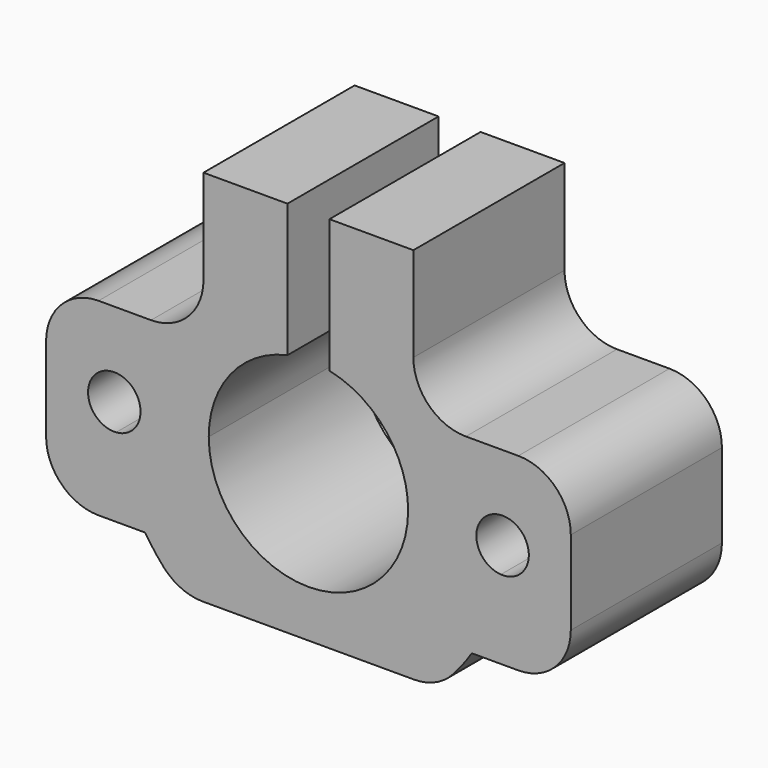
from build123d import *

# Parameters (mm, degrees)
F1_DEPTH = 18
F2_R     = 5


with BuildPart() as f1:
    # F0 (on Front) → F1 (new body)
    with BuildSketch(Plane.XZ):
        with BuildLine():
            ThreePointArc((12.0933866224, -14), (13.9727608958, -12.1248485743), (15.5643824163, -10))
            Line((15.5643824163, -10), (-15.5643824163, -10))
            ThreePointArc((-15.5643824163, -10), (-13.9727608958, -12.1248485743), (-12.0933866224, -14))
            Line((-12.0933866224, -14), (12.0933866224, -14))
        make_face()
        with BuildLine():
            Line((25, 8), (16.6808273176, 8))
            ThreePointArc((16.6808273176, 8), (17.7210793132, 5.311623855), (18.3310810811, 2.4942867515))
            ThreePointArc((18.3310810811, 2.4942867515), (20.2070006887, 1.8265127015), (21, 0))
            ThreePointArc((21, 0), (20.2070006887, -1.8265127015), (18.3310810811, -2.4942867515))
            ThreePointArc((18.3310810811, -2.4942867515), (17.358270198, -6.3984729219), (15.5643824163, -10))
            Line((15.5643824163, -10), (25, -10))
            Line((25, -10), (25, 8))
        make_face()
        with BuildLine():
            Line((2, 22), (2, 18.3915741577))
            ThreePointArc((2, 18.3915741577), (6.1642723241, 17.4428136123), (10, 15.5643824163))
            Line((10, 15.5643824163), (10, 22))
            Line((10, 22), (2, 22))
        make_face()
        with BuildLine():
            ThreePointArc((-10, 15.5643824163), (-6.1642723241, 17.4428136123), (-2, 18.3915741577))
            Line((-2, 18.3915741577), (-2, 22))
            Line((-2, 22), (-10, 22))
            Line((-10, 22), (-10, 15.5643824163))
        make_face()
        with BuildLine():
            ThreePointArc((-18.3310810811, 2.4942867515), (-17.7210793132, 5.311623855), (-16.6808273176, 8))
            Line((-16.6808273176, 8), (-25, 8))
            Line((-25, 8), (-25, -10))
            Line((-25, -10), (-15.5643824163, -10))
            ThreePointArc((-15.5643824163, -10), (-17.358270198, -6.3984729219), (-18.3310810811, -2.4942867515))
            ThreePointArc((-18.3310810811, -2.4942867515), (-21, 0), (-18.3310810811, 2.4942867515))
        make_face()
        with BuildLine():
            ThreePointArc((2, 9.2870878105), (3.6194093636, 8.7835002054), (5.123475383, 8))
            Line((5.123475383, 8), (10, 8))
            Line((10, 8), (10, 15.5643824163))
            ThreePointArc((10, 15.5643824163), (6.1642723241, 17.4428136123), (2, 18.3915741577))
            Line((2, 18.3915741577), (2, 9.2870878105))
        make_face()
        with BuildLine():
            Line((-10, 8), (-5.123475383, 8))
            ThreePointArc((-5.123475383, 8), (-3.6194093636, 8.7835002054), (-2, 9.2870878105))
            Line((-2, 9.2870878105), (-2, 18.3915741577))
            ThreePointArc((-2, 18.3915741577), (-6.1642723241, 17.4428136123), (-10, 15.5643824163))
            Line((-10, 15.5643824163), (-10, 8))
        make_face()
        with BuildLine():
            Line((10, 0), (9.5, 0))
            ThreePointArc((9.5, 0), (0, -9.5), (-9.5, 0))
            Line((-9.5, 0), (-10, 0))
            Line((-10, 0), (-10, 8))
            Line((-10, 8), (-16.6808273176, 8))
            ThreePointArc((-16.6808273176, 8), (-17.7210793132, 5.311623855), (-18.3310810811, 2.4942867515))
            ThreePointArc((-18.3310810811, 2.4942867515), (-16.6734872985, 1.7070006887), (-16, 0))
            ThreePointArc((-16, 0), (-16.6734872985, -1.7070006887), (-18.3310810811, -2.4942867515))
            ThreePointArc((-18.3310810811, -2.4942867515), (-17.358270198, -6.3984729219), (-15.5643824163, -10))
            Line((-15.5643824163, -10), (15.5643824163, -10))
            ThreePointArc((15.5643824163, -10), (17.358270198, -6.3984729219), (18.3310810811, -2.4942867515))
            ThreePointArc((18.3310810811, -2.4942867515), (16, 0), (18.3310810811, 2.4942867515))
            ThreePointArc((18.3310810811, 2.4942867515), (17.7210793132, 5.311623855), (16.6808273176, 8))
            Line((16.6808273176, 8), (10, 8))
            Line((10, 8), (10, 0))
        make_face()
        with BuildLine():
            Line((-10, 0), (-9.5, 0))
            ThreePointArc((-9.5, 0), (-8.3343570879, 4.5594398703), (-5.123475383, 8))
            Line((-5.123475383, 8), (-10, 8))
            Line((-10, 8), (-10, 0))
        make_face()
        with BuildLine():
            ThreePointArc((5.123475383, 8), (8.3343570879, 4.5594398703), (9.5, 0))
            Line((9.5, 0), (10, 0))
            Line((10, 0), (10, 8))
            Line((10, 8), (5.123475383, 8))
        make_face()
    extrude(amount=F1_DEPTH)

    # F2
    f2_edges = [f1.edges().sort_by_distance(p)[0] for p in [
        (-25, -9, 8),
        (-25, -9, -10),
        (25, -9, -10),
        (25, -9, 8),
        (10, -9, 8),
        (-10, -9, 8),
        (-12.093387, -9, -14),
        (12.093387, -9, -14),
    ]]
    fillet(f2_edges, radius=F2_R)


solid = f1.part
